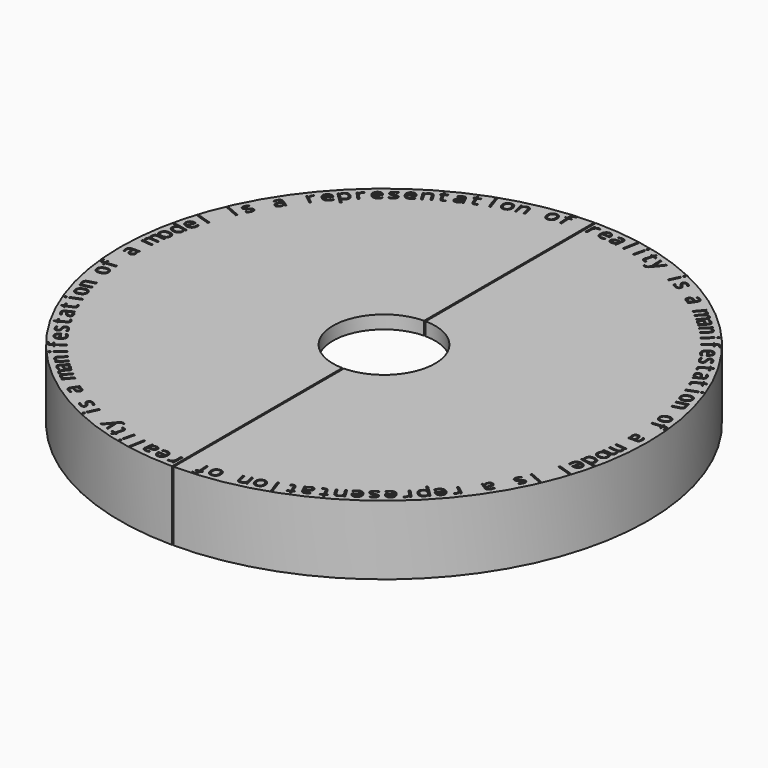
from build123d import *

# Parameters (mm, degrees)
F2_TEXT_SIZE  = 6.25
F3_DEPTH      = 0.5
F4_W          = 0.5
F4_H          = 250
F5_DEPTH      = 21.0010001
F6_R          = 1.125
F7_DEPTH      = 4.5
F7_DEPTH_BACK = 4.5


# Not quite as in the source:
# - Text() gives the source's letters only with a copy of the font that has no kerning and outlines rounded to 1/6400 em; it was checked with that copy


with BuildPart() as f1:
    # F0 (on Front) → F1 (revolve)
    with BuildSketch(Plane.XZ):
        Polygon((-76, 17), (-15.5, 17), (-15.5, 21), (-76, 21), (-80, 21), (-80, 0), (-76, 0), align=None)
    revolve(axis=Axis((0, 0, 4.5), (0, 0, 1)))

    # F2 (on face) → F3 (cut)
    with BuildSketch(Plane.XY.offset(21)):
        with Locations(Location((75, 1.6875), (0, 0, -90))):
            Text('a', F2_TEXT_SIZE, font='Open Sans', text_align=(TextAlign.LEFT, TextAlign.BOTTOM))
        with BuildLine():
            Line((76.5667712444, -9.8698071915), (74.4025219057, -9.6460911938))
            Line((74.4025219057, -9.6460911938), (74.3505089403, -10.1492694512))
            Line((74.3505089403, -10.1492694512), (75.2941063445, -10.2468080438))
            add(Edge.make_bspline(
                [(75.2941063445, -10.2468080438), (75.6206945725, -10.1947888387), (76.0030908282, -10.2543454638)],
                knots=[0.2674778804, 0.2674778804, 0.2674778804, 1, 1, 1], degree=2))
            add(Edge.make_bspline(
                [(76.0030908282, -10.2543454638), (76.257959575, -10.2940402101), (76.4710516616, -10.3684675454)],
                knots=[0, 0, 0, 0.3155698496, 0.3155698496, 0.3155698496], degree=2))
            Line((76.4710516616, -10.3684675454), (76.5205865986, -10.3735879156))
            add(Edge.make_bspline(
                [(77.4777653089, -10.1888000238), (77.1587875931, -10.4395580281), (76.5205865986, -10.3735879156)],
                knots=[0, 0, 0, 1, 1, 1], degree=2))
            add(Edge.make_bspline(
                [(77.8550818913, -9.3736664064), (77.7967430248, -9.9380420194), (77.4777653089, -10.1888000238)],
                knots=[0, 0, 0, 1, 1, 1], degree=2))
            add(Edge.make_bspline(
                [(77.7695822625, -8.7144084439), (77.8924348317, -9.0123105922), (77.8550818913, -9.3736664064)],
                knots=[0, 0, 0, 1, 1, 1], degree=2))
            add(Edge.make_bspline(
                [(77.4007896015, -8.2408735522), (77.6467296933, -8.4165062955), (77.7695822625, -8.7144084439)],
                knots=[0, 0, 0, 1, 1, 1], degree=2))
            Line((77.4007896015, -8.2408735522), (77.4032998798, -8.2165888872))
            add(Edge.make_bspline(
                [(78.0740785659, -7.2550722378), (77.9934484285, -8.0350956754), (77.4032998798, -8.2165888872)],
                knots=[0, 0, 0, 1, 1, 1], degree=2))
            add(Edge.make_bspline(
                [(77.997209117, -6.65953939), (78.1073146499, -6.9335432741), (78.0740785659, -7.2550722378)],
                knots=[0, 0, 0, 1, 1, 1], degree=2))
            add(Edge.make_bspline(
                [(77.6590173708, -6.2176388935), (77.887103584, -6.3855355059), (77.997209117, -6.65953939)],
                knots=[0, 0, 0, 1, 1, 1], degree=2))
            Line((77.6590173708, -6.2176388935), (77.6615276491, -6.1933542286))
            Line((77.6615276491, -6.1933542286), (78.1255424981, -6.1588505744))
            Line((78.1255424981, -6.1588505744), (78.167915995, -5.7489254304))
            Line((78.167915995, -5.7489254304), (74.8409168993, -5.4050173101))
            Line((74.8409168993, -5.4050173101), (74.7888035228, -5.909166954))
            Line((74.7888035228, -5.909166954), (76.5343852382, -6.0896057547))
            add(Edge.make_bspline(
                [(77.4422304774, -6.4058186815), (77.1813287119, -6.1564795673), (76.5343852382, -6.0896057547)],
                knots=[0, 0, 0, 1, 1, 1], degree=2))
            add(Edge.make_bspline(
                [(77.6542320225, -7.1282230687), (77.7031322429, -6.6551577958), (77.4422304774, -6.4058186815)],
                knots=[0, 0, 0, 1, 1, 1], degree=2))
            add(Edge.make_bspline(
                [(77.4006585753, -7.6390374613), (77.6168790822, -7.4895788828), (77.6542320225, -7.1282230687)],
                knots=[0, 0, 0, 1, 1, 1], degree=2))
            add(Edge.make_bspline(
                [(76.7861695635, -7.7473274764), (77.1844380684, -7.7884960397), (77.4006585753, -7.6390374613)],
                knots=[0, 0, 0, 1, 1, 1], degree=2))
            Line((76.7861695635, -7.7473274764), (74.6219202248, -7.5236114787))
            Line((74.6219202248, -7.5236114787), (74.5698068483, -8.0277611227))
            Line((74.5698068483, -8.0277611227), (76.4280694089, -8.2198476144))
            add(Edge.make_bspline(
                [(77.2363311595, -8.530675539), (76.9895308621, -8.2778852476), (76.4280694089, -8.2198476144)],
                knots=[0, 0, 0, 1, 1, 1], degree=2))
            add(Edge.make_bspline(
                [(77.4345324701, -9.2536169435), (77.483131457, -8.7834658304), (77.2363311595, -8.530675539)],
                knots=[0, 0, 0, 1, 1, 1], degree=2))
            add(Edge.make_bspline(
                [(77.1812602562, -9.7615171763), (77.3974807631, -9.6120585979), (77.4345324701, -9.2536169435)],
                knots=[0, 0, 0, 1, 1, 1], degree=2))
            add(Edge.make_bspline(
                [(76.5667712444, -9.8698071915), (76.9650397493, -9.9109757548), (77.1812602562, -9.7615171763)],
                knots=[0, 0, 0, 1, 1, 1], degree=2))
        make_face()
        with BuildLine():
            add(Edge.make_bspline(
                [(75.2941063445, -10.2468080438), (75.6206945725, -10.1947888387), (76.0030908282, -10.2543454638)],
                knots=[0.2674778804, 0.2674778804, 0.2674778804, 1, 1, 1], degree=2))
            Line((75.2941063445, -10.2468080438), (76.4710516616, -10.3684675454))
            add(Edge.make_bspline(
                [(76.0030908282, -10.2543454638), (76.257959575, -10.2940402101), (76.4710516616, -10.3684675454)],
                knots=[0, 0, 0, 0.3155698496, 0.3155698496, 0.3155698496], degree=2))
        make_face()
        with BuildLine():
            Line((76.4710516616, -10.3684675454), (75.2941063445, -10.2468080438))
            add(Edge.make_bspline(
                [(75.0630422483, -10.2996739281), (75.1748537996, -10.265802674), (75.2941063445, -10.2468080438)],
                knots=[0, 0, 0, 0.2674778804, 0.2674778804, 0.2674778804], degree=2))
            add(Edge.make_bspline(
                [(74.3830947631, -10.737359549), (74.6450205745, -10.4263059099), (75.0630422483, -10.2996739281)],
                knots=[0, 0, 0, 1, 1, 1], degree=2))
            add(Edge.make_bspline(
                [(74.0520384192, -11.4922807977), (74.1211689517, -11.0484131881), (74.3830947631, -10.737359549)],
                knots=[0, 0, 0, 1, 1, 1], degree=2))
            add(Edge.make_bspline(
                [(74.3308820598, -12.6876147423), (73.9402272971, -12.2101884097), (74.0520384192, -11.4922807977)],
                knots=[0, 0, 0, 1, 1, 1], degree=2))
            add(Edge.make_bspline(
                [(75.5301478156, -13.290978871), (74.7215368225, -13.1650410748), (74.3308820598, -12.6876147423)],
                knots=[0, 0, 0, 1, 1, 1], degree=2))
            add(Edge.make_bspline(
                [(76.8419294102, -13.076723243), (76.3165654282, -13.4134601405), (75.5301478156, -13.290978871)],
                knots=[0, 0, 0, 1, 1, 1], degree=2))
            add(Edge.make_bspline(
                [(77.4751971363, -12.0471669028), (77.3672933921, -12.7399863455), (76.8419294102, -13.076723243)],
                knots=[0, 0, 0, 1, 1, 1], degree=2))
            add(Edge.make_bspline(
                [(77.1988725751, -10.8546961335), (77.5870082585, -11.3292592908), (77.4751971363, -12.0471669028)],
                knots=[0, 0, 0, 1, 1, 1], degree=2))
            add(Edge.make_bspline(
                [(76.4710516616, -10.3684675454), (76.9332208109, -10.5298908003), (77.1988725751, -10.8546961335)],
                knots=[0.3155698496, 0.3155698496, 0.3155698496, 1, 1, 1], degree=2))
        make_face()
        with BuildLine():
            add(Edge.make_bspline(
                [(75.9222381619, -10.7734775811), (75.2882794239, -10.6747411466), (74.9173766224, -10.8764126892)],
                knots=[0, 0, 0, 1, 1, 1], degree=2))
            add(Edge.make_bspline(
                [(76.844791857, -11.1736345818), (76.5610215479, -10.8729654344), (75.9222381619, -10.7734775811)],
                knots=[0, 0, 0, 1, 1, 1], degree=2))
            add(Edge.make_bspline(
                [(77.0520677292, -11.9654528885), (77.1285621662, -11.4743037292), (76.844791857, -11.1736345818)],
                knots=[0, 0, 0, 1, 1, 1], degree=2))
            add(Edge.make_bspline(
                [(76.6077352618, -12.6671517688), (76.9745213057, -12.4633565548), (77.0520677292, -11.9654528885)],
                knots=[0, 0, 0, 1, 1, 1], degree=2))
            add(Edge.make_bspline(
                [(75.6108501981, -12.7728116833), (76.2409492178, -12.8709469827), (76.6077352618, -12.6671517688)],
                knots=[0, 0, 0, 1, 1, 1], degree=2))
            add(Edge.make_bspline(
                [(74.6836656672, -12.3674859387), (74.9739966713, -12.6736243975), (75.6108501981, -12.7728116833)],
                knots=[0, 0, 0, 1, 1, 1], degree=2))
            add(Edge.make_bspline(
                [(74.4699793839, -11.5692333911), (74.3933346631, -12.06134748), (74.6836656672, -12.3674859387)],
                knots=[0, 0, 0, 1, 1, 1], degree=2))
            add(Edge.make_bspline(
                [(74.9173766224, -10.8764126892), (74.546473821, -11.0780842318), (74.4699793839, -11.5692333911)],
                knots=[0, 0, 0, 1, 1, 1], degree=2))
        make_face(mode=Mode.SUBTRACT)
        with Locations(Location((73.7924179224, -13.5313822644), (0, 0, -101.8032786885))):
            Text('d', F2_TEXT_SIZE, font='Open Sans', text_align=(TextAlign.LEFT, TextAlign.BOTTOM))
        with Locations(Location((72.9835723683, -17.3669557087), (0, 0, -104.7540983607))):
            Text('e', F2_TEXT_SIZE, font='Open Sans', text_align=(TextAlign.LEFT, TextAlign.BOTTOM))
        with Locations(Location((71.6680180188, -22.1183238967), (0, 0, -107.7049180328))):
            Text('l', F2_TEXT_SIZE, font='Open Sans', text_align=(TextAlign.LEFT, TextAlign.BOTTOM))
        with Locations(Location((69.0237171975, -29.3477000862), (0, 0, -113.606557377))):
            Text('i', F2_TEXT_SIZE, font='Open Sans', text_align=(TextAlign.LEFT, TextAlign.BOTTOM))
        with Locations(Location((67.7794392233, -32.1457542009), (0, 0, -116.5573770492))):
            Text('s', F2_TEXT_SIZE, font='Open Sans', text_align=(TextAlign.LEFT, TextAlign.BOTTOM))
        with Locations(Location((64.1888418141, -38.8283432922), (0, 0, -122.4590163934))):
            Text('a', F2_TEXT_SIZE, font='Open Sans', text_align=(TextAlign.LEFT, TextAlign.BOTTOM))
        with Locations(Location((11.5285800565, -74.1333753891), (0, 0, -172.6229508197))):
            Text('o', F2_TEXT_SIZE, font='Open Sans', text_align=(TextAlign.LEFT, TextAlign.BOTTOM))
        with Locations(Location((55.068111233, -50.9537208547), (0, 0, -134.262295082))):
            Text('p', F2_TEXT_SIZE, font='Open Sans', text_align=(TextAlign.LEFT, TextAlign.BOTTOM))
        with Locations(Location((59.6989903996, -45.4212190121), (0, 0, -128.3606557377))):
            Text('r', F2_TEXT_SIZE, font='Open Sans', text_align=(TextAlign.LEFT, TextAlign.BOTTOM))
        with Locations(Location((57.518204598, -48.1650197348), (0, 0, -131.3114754098))):
            Text('e', F2_TEXT_SIZE, font='Open Sans', text_align=(TextAlign.LEFT, TextAlign.BOTTOM))
        with Locations(Location((51.9979522343, -54.0672687928), (0, 0, -137.2131147541))):
            Text('r', F2_TEXT_SIZE, font='Open Sans', text_align=(TextAlign.LEFT, TextAlign.BOTTOM))
        with Locations(Location((49.4208991042, -56.4427826915), (0, 0, -140.1639344262))):
            Text('e', F2_TEXT_SIZE, font='Open Sans', text_align=(TextAlign.LEFT, TextAlign.BOTTOM))
        with Locations(Location((46.2556656519, -59.05772845), (0, 0, -143.1147540984))):
            Text('s', F2_TEXT_SIZE, font='Open Sans', text_align=(TextAlign.LEFT, TextAlign.BOTTOM))
        with Locations(Location((40.211901713, -63.336376967), (0, 0, -149.0163934426))):
            Text('n', F2_TEXT_SIZE, font='Open Sans', text_align=(TextAlign.LEFT, TextAlign.BOTTOM))
        with Locations(Location((43.3554589942, -61.2251350479), (0, 0, -146.0655737705))):
            Text('e', F2_TEXT_SIZE, font='Open Sans', text_align=(TextAlign.LEFT, TextAlign.BOTTOM))
        with Locations(Location((36.3429843148, -65.6180285623), (0, 0, -151.9672131148))):
            Text('t', F2_TEXT_SIZE, font='Open Sans', text_align=(TextAlign.LEFT, TextAlign.BOTTOM))
        with Locations(Location((33.3219518722, -67.2123141967), (0, 0, -154.9180327869))):
            Text('a', F2_TEXT_SIZE, font='Open Sans', text_align=(TextAlign.LEFT, TextAlign.BOTTOM))
        with Locations(Location((29.4034508505, -69.0070667352), (0, 0, -157.868852459))):
            Text('t', F2_TEXT_SIZE, font='Open Sans', text_align=(TextAlign.LEFT, TextAlign.BOTTOM))
        with Locations(Location((25.3481232121, -70.5906062145), (0, 0, -160.8196721311))):
            Text('i', F2_TEXT_SIZE, font='Open Sans', text_align=(TextAlign.LEFT, TextAlign.BOTTOM))
        with Locations(Location((22.7996783046, -71.4761510848), (0, 0, -163.7704918033))):
            Text('o', F2_TEXT_SIZE, font='Open Sans', text_align=(TextAlign.LEFT, TextAlign.BOTTOM))
        with Locations(Location((7.1799922318, -74.66857784), (0, 0, -175.5737704918))):
            Text('f', F2_TEXT_SIZE, font='Open Sans', text_align=(TextAlign.LEFT, TextAlign.BOTTOM))
        with Locations(Location((19.0457486396, -72.5655093376), (0, 0, -166.7213114754))):
            Text('n', F2_TEXT_SIZE, font='Open Sans', text_align=(TextAlign.LEFT, TextAlign.BOTTOM))
        with Locations(Location((-0.4974869377, -75.0120596839), (0, 0, 178.5245901639))):
            Text('r', F2_TEXT_SIZE, font='Open Sans', text_align=(TextAlign.LEFT, TextAlign.BOTTOM))
        with Locations(Location((-4.0010252163, -74.9146499922), (0, 0, 175.5737704918))):
            Text('e', F2_TEXT_SIZE, font='Open Sans', text_align=(TextAlign.LEFT, TextAlign.BOTTOM))
        with Locations(Location((-7.9563446234, -74.5958727845), (0, 0, 172.6229508197))):
            Text('a', F2_TEXT_SIZE, font='Open Sans', text_align=(TextAlign.LEFT, TextAlign.BOTTOM))
        with Locations(Location((-12.733187692, -73.9147548866), (0, 0, 169.6721311475))):
            Text('l', F2_TEXT_SIZE, font='Open Sans', text_align=(TextAlign.LEFT, TextAlign.BOTTOM))
        with Locations(Location((-16.4975828331, -73.1668695297), (0, 0, 166.7213114754))):
            Text('i', F2_TEXT_SIZE, font='Open Sans', text_align=(TextAlign.LEFT, TextAlign.BOTTOM))
        with Locations(Location((-19.7706117354, -72.357868217), (0, 0, 163.7704918033))):
            Text('t', F2_TEXT_SIZE, font='Open Sans', text_align=(TextAlign.LEFT, TextAlign.BOTTOM))
        with Locations(Location((-22.9647636739, -71.4196623814), (0, 0, 160.8196721311))):
            Text('y', F2_TEXT_SIZE, font='Open Sans', text_align=(TextAlign.LEFT, TextAlign.BOTTOM))
        with Locations(Location((-31.1151870808, -68.2451915452), (0, 0, 154.9180327869))):
            Text('i', F2_TEXT_SIZE, font='Open Sans', text_align=(TextAlign.LEFT, TextAlign.BOTTOM))
        with Locations(Location((-33.8802759878, -66.9292820338), (0, 0, 151.9672131148))):
            Text('s', F2_TEXT_SIZE, font='Open Sans', text_align=(TextAlign.LEFT, TextAlign.BOTTOM))
        with Locations(Location((-40.4681991916, -63.1678122974), (0, 0, 146.0655737705))):
            Text('a', F2_TEXT_SIZE, font='Open Sans', text_align=(TextAlign.LEFT, TextAlign.BOTTOM))
        with Locations(Location((-45.8514548433, -59.4205400456), (0, 0, 140.1639344262))):
            Text('m', F2_TEXT_SIZE, font='Open Sans', text_align=(TextAlign.LEFT, TextAlign.BOTTOM))
        with Locations(Location((-49.7070688614, -56.1876762418), (0, 0, 137.2131147541))):
            Text('a', F2_TEXT_SIZE, font='Open Sans', text_align=(TextAlign.LEFT, TextAlign.BOTTOM))
        with Locations(Location((-52.4068583499, -53.6844007563), (0, 0, 134.262295082))):
            Text('n', F2_TEXT_SIZE, font='Open Sans', text_align=(TextAlign.LEFT, TextAlign.BOTTOM))
        with Locations(Location((-55.8404254046, -50.0740244712), (0, 0, 131.3114754098))):
            Text('i', F2_TEXT_SIZE, font='Open Sans', text_align=(TextAlign.LEFT, TextAlign.BOTTOM))
        with Locations(Location((-57.9426170809, -47.6403393241), (0, 0, 128.3606557377))):
            Text('f', F2_TEXT_SIZE, font='Open Sans', text_align=(TextAlign.LEFT, TextAlign.BOTTOM))
        with Locations(Location((-60.088524312, -44.9175047418), (0, 0, 125.4098360656))):
            Text('e', F2_TEXT_SIZE, font='Open Sans', text_align=(TextAlign.LEFT, TextAlign.BOTTOM))
        with Locations(Location((-62.4513927095, -41.5599018672), (0, 0, 122.4590163934))):
            Text('s', F2_TEXT_SIZE, font='Open Sans', text_align=(TextAlign.LEFT, TextAlign.BOTTOM))
        with Locations(Location((-64.660518032, -38.0204627685), (0, 0, 119.5081967213))):
            Text('t', F2_TEXT_SIZE, font='Open Sans', text_align=(TextAlign.LEFT, TextAlign.BOTTOM))
        with Locations(Location((-66.3320603915, -35.0414814251), (0, 0, 116.5573770492))):
            Text('a', F2_TEXT_SIZE, font='Open Sans', text_align=(TextAlign.LEFT, TextAlign.BOTTOM))
        with Locations(Location((-68.2271111371, -31.1704906472), (0, 0, 113.606557377))):
            Text('t', F2_TEXT_SIZE, font='Open Sans', text_align=(TextAlign.LEFT, TextAlign.BOTTOM))
        with Locations(Location((-69.9145418476, -27.1572803195), (0, 0, 110.6557377049))):
            Text('i', F2_TEXT_SIZE, font='Open Sans', text_align=(TextAlign.LEFT, TextAlign.BOTTOM))
        with Locations(Location((-70.8654102704, -24.6324812371), (0, 0, 107.7049180328))):
            Text('o', F2_TEXT_SIZE, font='Open Sans', text_align=(TextAlign.LEFT, TextAlign.BOTTOM))
        with Locations(Location((-72.0510632225, -20.907844824), (0, 0, 104.7540983607))):
            Text('n', F2_TEXT_SIZE, font='Open Sans', text_align=(TextAlign.LEFT, TextAlign.BOTTOM))
        with Locations(Location((-73.811960883, -13.4335377062), (0, 0, 98.8524590164))):
            Text('o', F2_TEXT_SIZE, font='Open Sans', text_align=(TextAlign.LEFT, TextAlign.BOTTOM))
        with Locations(Location((-74.4589529607, -9.1001719261), (0, 0, 95.9016393443))):
            Text('f', F2_TEXT_SIZE, font='Open Sans', text_align=(TextAlign.LEFT, TextAlign.BOTTOM))
        with Locations(Location((-75, -1.6875), (0, 0, 90))):
            Text('a', F2_TEXT_SIZE, font='Open Sans', text_align=(TextAlign.LEFT, TextAlign.BOTTOM))
        with BuildLine():
            Line((-76.5667712444, 9.8698071915), (-74.4025219057, 9.6460911938))
            Line((-74.4025219057, 9.6460911938), (-74.3505089403, 10.1492694512))
            Line((-74.3505089403, 10.1492694512), (-75.2941063445, 10.2468080438))
            add(Edge.make_bspline(
                [(-75.2941063445, 10.2468080438), (-75.6206945725, 10.1947888387), (-76.0030908282, 10.2543454638)],
                knots=[0.2674778804, 0.2674778804, 0.2674778804, 1, 1, 1], degree=2))
            add(Edge.make_bspline(
                [(-76.0030908282, 10.2543454638), (-76.257959575, 10.2940402101), (-76.4710516616, 10.3684675454)],
                knots=[0, 0, 0, 0.3155698496, 0.3155698496, 0.3155698496], degree=2))
            Line((-76.4710516616, 10.3684675454), (-76.5205865986, 10.3735879156))
            add(Edge.make_bspline(
                [(-77.4777653089, 10.1888000238), (-77.1587875931, 10.4395580281), (-76.5205865986, 10.3735879156)],
                knots=[0, 0, 0, 1, 1, 1], degree=2))
            add(Edge.make_bspline(
                [(-77.8550818913, 9.3736664064), (-77.7967430248, 9.9380420194), (-77.4777653089, 10.1888000238)],
                knots=[0, 0, 0, 1, 1, 1], degree=2))
            add(Edge.make_bspline(
                [(-77.7695822625, 8.7144084439), (-77.8924348317, 9.0123105922), (-77.8550818913, 9.3736664064)],
                knots=[0, 0, 0, 1, 1, 1], degree=2))
            add(Edge.make_bspline(
                [(-77.4007896015, 8.2408735522), (-77.6467296933, 8.4165062955), (-77.7695822625, 8.7144084439)],
                knots=[0, 0, 0, 1, 1, 1], degree=2))
            Line((-77.4007896015, 8.2408735522), (-77.4032998798, 8.2165888872))
            add(Edge.make_bspline(
                [(-78.0740785659, 7.2550722378), (-77.9934484285, 8.0350956754), (-77.4032998798, 8.2165888872)],
                knots=[0, 0, 0, 1, 1, 1], degree=2))
            add(Edge.make_bspline(
                [(-77.997209117, 6.65953939), (-78.1073146499, 6.9335432741), (-78.0740785659, 7.2550722378)],
                knots=[0, 0, 0, 1, 1, 1], degree=2))
            add(Edge.make_bspline(
                [(-77.6590173708, 6.2176388935), (-77.887103584, 6.3855355059), (-77.997209117, 6.65953939)],
                knots=[0, 0, 0, 1, 1, 1], degree=2))
            Line((-77.6590173708, 6.2176388935), (-77.6615276491, 6.1933542286))
            Line((-77.6615276491, 6.1933542286), (-78.1255424981, 6.1588505744))
            Line((-78.1255424981, 6.1588505744), (-78.167915995, 5.7489254304))
            Line((-78.167915995, 5.7489254304), (-74.8409168993, 5.4050173101))
            Line((-74.8409168993, 5.4050173101), (-74.7888035228, 5.909166954))
            Line((-74.7888035228, 5.909166954), (-76.5343852382, 6.0896057547))
            add(Edge.make_bspline(
                [(-77.4422304774, 6.4058186815), (-77.1813287119, 6.1564795673), (-76.5343852382, 6.0896057547)],
                knots=[0, 0, 0, 1, 1, 1], degree=2))
            add(Edge.make_bspline(
                [(-77.6542320225, 7.1282230687), (-77.7031322429, 6.6551577958), (-77.4422304774, 6.4058186815)],
                knots=[0, 0, 0, 1, 1, 1], degree=2))
            add(Edge.make_bspline(
                [(-77.4006585753, 7.6390374613), (-77.6168790822, 7.4895788828), (-77.6542320225, 7.1282230687)],
                knots=[0, 0, 0, 1, 1, 1], degree=2))
            add(Edge.make_bspline(
                [(-76.7861695635, 7.7473274764), (-77.1844380684, 7.7884960397), (-77.4006585753, 7.6390374613)],
                knots=[0, 0, 0, 1, 1, 1], degree=2))
            Line((-76.7861695635, 7.7473274764), (-74.6219202248, 7.5236114787))
            Line((-74.6219202248, 7.5236114787), (-74.5698068483, 8.0277611227))
            Line((-74.5698068483, 8.0277611227), (-76.4280694089, 8.2198476144))
            add(Edge.make_bspline(
                [(-77.2363311595, 8.530675539), (-76.9895308621, 8.2778852476), (-76.4280694089, 8.2198476144)],
                knots=[0, 0, 0, 1, 1, 1], degree=2))
            add(Edge.make_bspline(
                [(-77.4345324701, 9.2536169435), (-77.483131457, 8.7834658304), (-77.2363311595, 8.530675539)],
                knots=[0, 0, 0, 1, 1, 1], degree=2))
            add(Edge.make_bspline(
                [(-77.1812602562, 9.7615171763), (-77.3974807631, 9.6120585979), (-77.4345324701, 9.2536169435)],
                knots=[0, 0, 0, 1, 1, 1], degree=2))
            add(Edge.make_bspline(
                [(-76.5667712444, 9.8698071915), (-76.9650397493, 9.9109757548), (-77.1812602562, 9.7615171763)],
                knots=[0, 0, 0, 1, 1, 1], degree=2))
        make_face()
        with BuildLine():
            add(Edge.make_bspline(
                [(-75.2941063445, 10.2468080438), (-75.6206945725, 10.1947888387), (-76.0030908282, 10.2543454638)],
                knots=[0.2674778804, 0.2674778804, 0.2674778804, 1, 1, 1], degree=2))
            Line((-75.2941063445, 10.2468080438), (-76.4710516616, 10.3684675454))
            add(Edge.make_bspline(
                [(-76.0030908282, 10.2543454638), (-76.257959575, 10.2940402101), (-76.4710516616, 10.3684675454)],
                knots=[0, 0, 0, 0.3155698496, 0.3155698496, 0.3155698496], degree=2))
        make_face()
        with BuildLine():
            Line((-76.4710516616, 10.3684675454), (-75.2941063445, 10.2468080438))
            add(Edge.make_bspline(
                [(-75.0630422483, 10.2996739281), (-75.1748537996, 10.265802674), (-75.2941063445, 10.2468080438)],
                knots=[0, 0, 0, 0.2674778804, 0.2674778804, 0.2674778804], degree=2))
            add(Edge.make_bspline(
                [(-74.3830947631, 10.737359549), (-74.6450205745, 10.4263059099), (-75.0630422483, 10.2996739281)],
                knots=[0, 0, 0, 1, 1, 1], degree=2))
            add(Edge.make_bspline(
                [(-74.0520384192, 11.4922807977), (-74.1211689517, 11.0484131881), (-74.3830947631, 10.737359549)],
                knots=[0, 0, 0, 1, 1, 1], degree=2))
            add(Edge.make_bspline(
                [(-74.3308820598, 12.6876147423), (-73.9402272971, 12.2101884097), (-74.0520384192, 11.4922807977)],
                knots=[0, 0, 0, 1, 1, 1], degree=2))
            add(Edge.make_bspline(
                [(-75.5301478156, 13.290978871), (-74.7215368225, 13.1650410748), (-74.3308820598, 12.6876147423)],
                knots=[0, 0, 0, 1, 1, 1], degree=2))
            add(Edge.make_bspline(
                [(-76.8419294102, 13.076723243), (-76.3165654282, 13.4134601405), (-75.5301478156, 13.290978871)],
                knots=[0, 0, 0, 1, 1, 1], degree=2))
            add(Edge.make_bspline(
                [(-77.4751971363, 12.0471669028), (-77.3672933921, 12.7399863455), (-76.8419294102, 13.076723243)],
                knots=[0, 0, 0, 1, 1, 1], degree=2))
            add(Edge.make_bspline(
                [(-77.1988725751, 10.8546961335), (-77.5870082585, 11.3292592908), (-77.4751971363, 12.0471669028)],
                knots=[0, 0, 0, 1, 1, 1], degree=2))
            add(Edge.make_bspline(
                [(-76.4710516616, 10.3684675454), (-76.9332208109, 10.5298908003), (-77.1988725751, 10.8546961335)],
                knots=[0.3155698496, 0.3155698496, 0.3155698496, 1, 1, 1], degree=2))
        make_face()
        with BuildLine():
            add(Edge.make_bspline(
                [(-75.9222381619, 10.7734775811), (-75.2882794239, 10.6747411466), (-74.9173766224, 10.8764126892)],
                knots=[0, 0, 0, 1, 1, 1], degree=2))
            add(Edge.make_bspline(
                [(-76.844791857, 11.1736345818), (-76.5610215479, 10.8729654344), (-75.9222381619, 10.7734775811)],
                knots=[0, 0, 0, 1, 1, 1], degree=2))
            add(Edge.make_bspline(
                [(-77.0520677292, 11.9654528885), (-77.1285621662, 11.4743037292), (-76.844791857, 11.1736345818)],
                knots=[0, 0, 0, 1, 1, 1], degree=2))
            add(Edge.make_bspline(
                [(-76.6077352618, 12.6671517688), (-76.9745213057, 12.4633565548), (-77.0520677292, 11.9654528885)],
                knots=[0, 0, 0, 1, 1, 1], degree=2))
            add(Edge.make_bspline(
                [(-75.6108501981, 12.7728116833), (-76.2409492178, 12.8709469827), (-76.6077352618, 12.6671517688)],
                knots=[0, 0, 0, 1, 1, 1], degree=2))
            add(Edge.make_bspline(
                [(-74.6836656672, 12.3674859387), (-74.9739966713, 12.6736243975), (-75.6108501981, 12.7728116833)],
                knots=[0, 0, 0, 1, 1, 1], degree=2))
            add(Edge.make_bspline(
                [(-74.4699793839, 11.5692333911), (-74.3933346631, 12.06134748), (-74.6836656672, 12.3674859387)],
                knots=[0, 0, 0, 1, 1, 1], degree=2))
            add(Edge.make_bspline(
                [(-74.9173766224, 10.8764126892), (-74.546473821, 11.0780842318), (-74.4699793839, 11.5692333911)],
                knots=[0, 0, 0, 1, 1, 1], degree=2))
        make_face(mode=Mode.SUBTRACT)
        with Locations(Location((-73.7924179224, 13.5313822644), (0, 0, 78.1967213115))):
            Text('d', F2_TEXT_SIZE, font='Open Sans', text_align=(TextAlign.LEFT, TextAlign.BOTTOM))
        with Locations(Location((-72.9835723683, 17.3669557087), (0, 0, 75.2459016393))):
            Text('e', F2_TEXT_SIZE, font='Open Sans', text_align=(TextAlign.LEFT, TextAlign.BOTTOM))
        with Locations(Location((-71.6680180188, 22.1183238967), (0, 0, 72.2950819672))):
            Text('l', F2_TEXT_SIZE, font='Open Sans', text_align=(TextAlign.LEFT, TextAlign.BOTTOM))
        with Locations(Location((-69.0237171975, 29.3477000862), (0, 0, 66.393442623))):
            Text('i', F2_TEXT_SIZE, font='Open Sans', text_align=(TextAlign.LEFT, TextAlign.BOTTOM))
        with Locations(Location((-67.7794392233, 32.1457542009), (0, 0, 63.4426229508))):
            Text('s', F2_TEXT_SIZE, font='Open Sans', text_align=(TextAlign.LEFT, TextAlign.BOTTOM))
        with Locations(Location((-64.1888418141, 38.8283432922), (0, 0, 57.5409836066))):
            Text('a', F2_TEXT_SIZE, font='Open Sans', text_align=(TextAlign.LEFT, TextAlign.BOTTOM))
        with Locations(Location((-59.6989903996, 45.4212190121), (0, 0, 51.6393442623))):
            Text('r', F2_TEXT_SIZE, font='Open Sans', text_align=(TextAlign.LEFT, TextAlign.BOTTOM))
        with Locations(Location((-57.518204598, 48.1650197348), (0, 0, 48.6885245902))):
            Text('e', F2_TEXT_SIZE, font='Open Sans', text_align=(TextAlign.LEFT, TextAlign.BOTTOM))
        with Locations(Location((-55.068111233, 50.9537208547), (0, 0, 45.737704918))):
            Text('p', F2_TEXT_SIZE, font='Open Sans', text_align=(TextAlign.LEFT, TextAlign.BOTTOM))
        with Locations(Location((-51.9979522343, 54.0672687928), (0, 0, 42.7868852459))):
            Text('r', F2_TEXT_SIZE, font='Open Sans', text_align=(TextAlign.LEFT, TextAlign.BOTTOM))
        with Locations(Location((-49.4208991042, 56.4427826915), (0, 0, 39.8360655738))):
            Text('e', F2_TEXT_SIZE, font='Open Sans', text_align=(TextAlign.LEFT, TextAlign.BOTTOM))
        with Locations(Location((-46.2556656519, 59.05772845), (0, 0, 36.8852459016))):
            Text('s', F2_TEXT_SIZE, font='Open Sans', text_align=(TextAlign.LEFT, TextAlign.BOTTOM))
        with Locations(Location((-43.3554589942, 61.2251350479), (0, 0, 33.9344262295))):
            Text('e', F2_TEXT_SIZE, font='Open Sans', text_align=(TextAlign.LEFT, TextAlign.BOTTOM))
        with Locations(Location((-40.211901713, 63.336376967), (0, 0, 30.9836065574))):
            Text('n', F2_TEXT_SIZE, font='Open Sans', text_align=(TextAlign.LEFT, TextAlign.BOTTOM))
        with Locations(Location((-36.3429843148, 65.6180285623), (0, 0, 28.0327868852))):
            Text('t', F2_TEXT_SIZE, font='Open Sans', text_align=(TextAlign.LEFT, TextAlign.BOTTOM))
        with Locations(Location((-33.3219518722, 67.2123141967), (0, 0, 25.0819672131))):
            Text('a', F2_TEXT_SIZE, font='Open Sans', text_align=(TextAlign.LEFT, TextAlign.BOTTOM))
        with Locations(Location((-29.4034508505, 69.0070667352), (0, 0, 22.131147541))):
            Text('t', F2_TEXT_SIZE, font='Open Sans', text_align=(TextAlign.LEFT, TextAlign.BOTTOM))
        with Locations(Location((-25.3481232121, 70.5906062145), (0, 0, 19.1803278689))):
            Text('i', F2_TEXT_SIZE, font='Open Sans', text_align=(TextAlign.LEFT, TextAlign.BOTTOM))
        with Locations(Location((-22.7996783046, 71.4761510848), (0, 0, 16.2295081967))):
            Text('o', F2_TEXT_SIZE, font='Open Sans', text_align=(TextAlign.LEFT, TextAlign.BOTTOM))
        with Locations(Location((-19.0457486396, 72.5655093376), (0, 0, 13.2786885246))):
            Text('n', F2_TEXT_SIZE, font='Open Sans', text_align=(TextAlign.LEFT, TextAlign.BOTTOM))
        with Locations(Location((-11.5285800565, 74.1333753891), (0, 0, 7.3770491803))):
            Text('o', F2_TEXT_SIZE, font='Open Sans', text_align=(TextAlign.LEFT, TextAlign.BOTTOM))
        with Locations(Location((-7.1799922318, 74.66857784), (0, 0, 4.4262295082))):
            Text('f', F2_TEXT_SIZE, font='Open Sans', text_align=(TextAlign.LEFT, TextAlign.BOTTOM))
        with Locations(Location((0.4974869377, 75.0120596839), (0, 0, -1.4754098361))):
            Text('r', F2_TEXT_SIZE, font='Open Sans', text_align=(TextAlign.LEFT, TextAlign.BOTTOM))
        with Locations(Location((4.0010252163, 74.9146499922), (0, 0, -4.4262295082))):
            Text('e', F2_TEXT_SIZE, font='Open Sans', text_align=(TextAlign.LEFT, TextAlign.BOTTOM))
        with Locations(Location((7.9563446234, 74.5958727845), (0, 0, -7.3770491803))):
            Text('a', F2_TEXT_SIZE, font='Open Sans', text_align=(TextAlign.LEFT, TextAlign.BOTTOM))
        with Locations(Location((12.733187692, 73.9147548866), (0, 0, -10.3278688525))):
            Text('l', F2_TEXT_SIZE, font='Open Sans', text_align=(TextAlign.LEFT, TextAlign.BOTTOM))
        with Locations(Location((16.4975828331, 73.1668695297), (0, 0, -13.2786885246))):
            Text('i', F2_TEXT_SIZE, font='Open Sans', text_align=(TextAlign.LEFT, TextAlign.BOTTOM))
        with Locations(Location((19.7706117354, 72.357868217), (0, 0, -16.2295081967))):
            Text('t', F2_TEXT_SIZE, font='Open Sans', text_align=(TextAlign.LEFT, TextAlign.BOTTOM))
        with Locations(Location((22.9647636739, 71.4196623814), (0, 0, -19.1803278689))):
            Text('y', F2_TEXT_SIZE, font='Open Sans', text_align=(TextAlign.LEFT, TextAlign.BOTTOM))
        with Locations(Location((31.1151870808, 68.2451915452), (0, 0, -25.0819672131))):
            Text('i', F2_TEXT_SIZE, font='Open Sans', text_align=(TextAlign.LEFT, TextAlign.BOTTOM))
        with Locations(Location((33.8802759878, 66.9292820338), (0, 0, -28.0327868852))):
            Text('s', F2_TEXT_SIZE, font='Open Sans', text_align=(TextAlign.LEFT, TextAlign.BOTTOM))
        with Locations(Location((40.4681991916, 63.1678122974), (0, 0, -33.9344262295))):
            Text('a', F2_TEXT_SIZE, font='Open Sans', text_align=(TextAlign.LEFT, TextAlign.BOTTOM))
        with Locations(Location((45.8514548433, 59.4205400456), (0, 0, -39.8360655738))):
            Text('m', F2_TEXT_SIZE, font='Open Sans', text_align=(TextAlign.LEFT, TextAlign.BOTTOM))
        with Locations(Location((49.7070688614, 56.1876762418), (0, 0, -42.7868852459))):
            Text('a', F2_TEXT_SIZE, font='Open Sans', text_align=(TextAlign.LEFT, TextAlign.BOTTOM))
        with Locations(Location((52.4068583499, 53.6844007563), (0, 0, -45.737704918))):
            Text('n', F2_TEXT_SIZE, font='Open Sans', text_align=(TextAlign.LEFT, TextAlign.BOTTOM))
        with Locations(Location((55.8404254046, 50.0740244712), (0, 0, -48.6885245902))):
            Text('i', F2_TEXT_SIZE, font='Open Sans', text_align=(TextAlign.LEFT, TextAlign.BOTTOM))
        with Locations(Location((57.9426170809, 47.6403393241), (0, 0, -51.6393442623))):
            Text('f', F2_TEXT_SIZE, font='Open Sans', text_align=(TextAlign.LEFT, TextAlign.BOTTOM))
        with Locations(Location((60.088524312, 44.9175047418), (0, 0, -54.5901639344))):
            Text('e', F2_TEXT_SIZE, font='Open Sans', text_align=(TextAlign.LEFT, TextAlign.BOTTOM))
        with Locations(Location((62.4513927095, 41.5599018672), (0, 0, -57.5409836066))):
            Text('s', F2_TEXT_SIZE, font='Open Sans', text_align=(TextAlign.LEFT, TextAlign.BOTTOM))
        with Locations(Location((64.660518032, 38.0204627685), (0, 0, -60.4918032787))):
            Text('t', F2_TEXT_SIZE, font='Open Sans', text_align=(TextAlign.LEFT, TextAlign.BOTTOM))
        with Locations(Location((66.3320603915, 35.0414814251), (0, 0, -63.4426229508))):
            Text('a', F2_TEXT_SIZE, font='Open Sans', text_align=(TextAlign.LEFT, TextAlign.BOTTOM))
        with Locations(Location((68.2271111371, 31.1704906472), (0, 0, -66.393442623))):
            Text('t', F2_TEXT_SIZE, font='Open Sans', text_align=(TextAlign.LEFT, TextAlign.BOTTOM))
        with Locations(Location((69.9145418476, 27.1572803195), (0, 0, -69.3442622951))):
            Text('i', F2_TEXT_SIZE, font='Open Sans', text_align=(TextAlign.LEFT, TextAlign.BOTTOM))
        with Locations(Location((70.8654102704, 24.6324812371), (0, 0, -72.2950819672))):
            Text('o', F2_TEXT_SIZE, font='Open Sans', text_align=(TextAlign.LEFT, TextAlign.BOTTOM))
        with Locations(Location((72.0510632225, 20.907844824), (0, 0, -75.2459016393))):
            Text('n', F2_TEXT_SIZE, font='Open Sans', text_align=(TextAlign.LEFT, TextAlign.BOTTOM))
        with Locations(Location((73.811960883, 13.4335377062), (0, 0, -81.1475409836))):
            Text('o', F2_TEXT_SIZE, font='Open Sans', text_align=(TextAlign.LEFT, TextAlign.BOTTOM))
        with Locations(Location((74.4589529607, 9.1001719261), (0, 0, -84.0983606557))):
            Text('f', F2_TEXT_SIZE, font='Open Sans', text_align=(TextAlign.LEFT, TextAlign.BOTTOM))
    extrude(amount=-F3_DEPTH, mode=Mode.SUBTRACT)

    # F4 (on Top) → F5 (cut, through all)
    with BuildSketch(Plane.XY):
        Rectangle(F4_W, F4_H)
    extrude(amount=F5_DEPTH, mode=Mode.SUBTRACT)

    # F6 (on Right) → F7 (cut, two sides)
    with BuildSketch(Plane.YZ) as f7_sk:
        with Locations((78, 19)):
            Circle(F6_R)
        with Locations((78, 2)):
            Circle(F6_R)
        with Locations((-78, 19)):
            Circle(F6_R)
        with Locations((-78, 2)):
            Circle(F6_R)
    extrude(amount=F7_DEPTH, mode=Mode.SUBTRACT)
    extrude(f7_sk.sketch, amount=-F7_DEPTH_BACK, mode=Mode.SUBTRACT)


solid = f1.part
